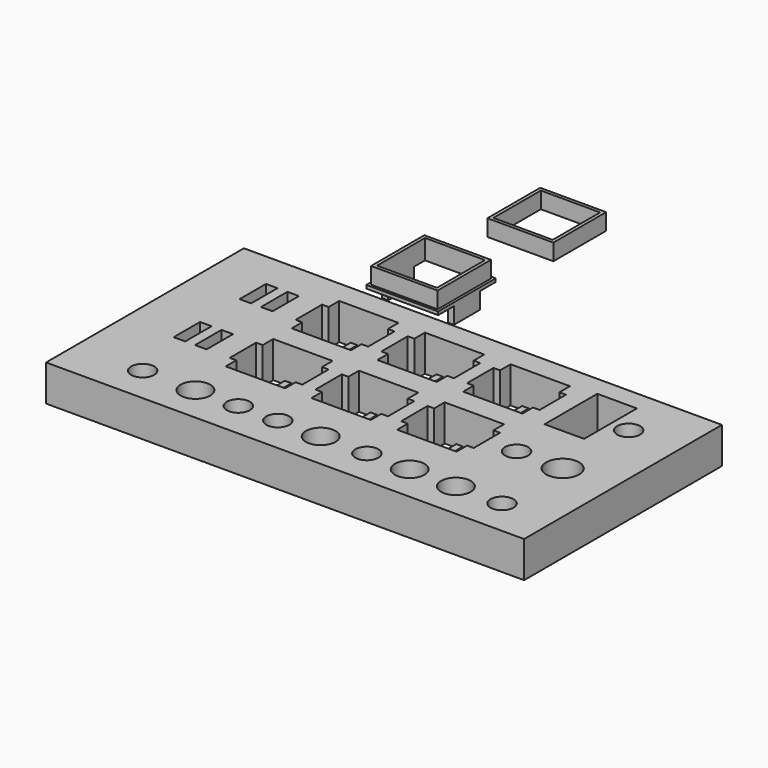
from build123d import *

# Parameters (mm, degrees)
F0_W      = 145
F0_H      = 75
F0_R      = 3.5
F0_R_2    = 4.5
F0_R_3    = 5
F0_W_2    = 12
F0_H_2    = 20
F0_W_3    = 3
F0_H_3    = 10
F1_DEPTH  = 1
F2_DEPTH  = 10
F3_W      = 18
F3_H      = 18
F4_DEPTH  = 10
F5_W      = 2
F5_H      = 10
F6_DEPTH  = 10
F8_DEPTH  = 5
F7_W      = 1.8
F7_H      = 9.8
F9_DEPTH  = 1
F10_DEPTH = 5
F11_W     = 20.2
F11_H     = 20.2
F11_W_2   = 18.2
F11_H_2   = 18.2
F12_DEPTH = 5


with BuildPart() as f1:
    # F0 (on Top) → F1 (new body)
    with BuildSketch(Plane.XY):
        with Locations((-82.504784634, -17.5405644029)):
            Rectangle(F0_W, F0_H)
        with Locations((-134.504784634, -44.0405644029)):
            Circle(F0_R, mode=Mode.SUBTRACT)
        with Locations((-118.504784634, -44.0405644029)):
            Circle(F0_R_2, mode=Mode.SUBTRACT)
        with Locations((-105.504784634, -44.0405644029)):
            Circle(F0_R, mode=Mode.SUBTRACT)
        with Locations((-93.504784634, -44.0405644029)):
            Circle(F0_R, mode=Mode.SUBTRACT)
        Polygon((-129.504784634, -16.0405644029), (-129.504784634, -26.0405644029), (-133.004784634, -26.0405644029), (-136.004784634, -26.0405644029), (-139.504784634, -26.0405644029), (-139.504784634, -16.0405644029), (-136.004784634, -16.0405644029), (-133.004784634, -16.0405644029), align=None, mode=Mode.SUBTRACT)
        Polygon((-102.504784634, -22.0405644029), (-102.504784634, -30.0405644029), (-105.9770819313, -30.0405644029), (-107.9770819313, -30.0405644029), (-114.9770819313, -30.0405644029), (-116.9770819313, -30.0405644029), (-120.504784634, -30.0405644029), (-120.504784634, -22.0405644029), (-120.504784634, -20.0405644029), (-120.504784634, -12.0405644029), (-116.9770819313, -12.0405644029), (-114.9770819313, -12.0405644029), (-107.9770819313, -12.0405644029), (-105.9770819313, -12.0405644029), (-102.504784634, -12.0405644029), (-102.504784634, -20.0405644029), align=None, mode=Mode.SUBTRACT)
        Polygon((-76.504784634, -12.0405644029), (-76.504784634, -20.0405644029), (-76.504784634, -22.0405644029), (-76.504784634, -30.0405644029), (-79.9770819313, -30.0405644029), (-81.9770819313, -30.0405644029), (-88.9770819313, -30.0405644029), (-90.9770819313, -30.0405644029), (-94.504784634, -30.0405644029), (-94.504784634, -22.0405644029), (-94.504784634, -20.0405644029), (-94.504784634, -12.0405644029), (-90.9770819313, -12.0405644029), (-88.9770819313, -12.0405644029), (-81.9770819313, -12.0405644029), (-79.9770819313, -12.0405644029), align=None, mode=Mode.SUBTRACT)
        with Locations((-80.504784634, -44.0405644029)):
            Circle(F0_R_2, mode=Mode.SUBTRACT)
        with Locations((-66.504784634, -44.0405644029)):
            Circle(F0_R, mode=Mode.SUBTRACT)
        with Locations((-53.504784634, -44.0405644029)):
            Circle(F0_R_2, mode=Mode.SUBTRACT)
        with Locations((-39.504784634, -44.0405644029)):
            Circle(F0_R_2, mode=Mode.SUBTRACT)
        with Locations((-25.504784634, -44.0405644029)):
            Circle(F0_R, mode=Mode.SUBTRACT)
        Polygon((-50.504784634, -12.0405644029), (-50.504784634, -20.0405644029), (-50.504784634, -22.0405644029), (-50.504784634, -30.0405644029), (-53.9770819313, -30.0405644029), (-55.9770819313, -30.0405644029), (-62.9770819313, -30.0405644029), (-64.9770819313, -30.0405644029), (-68.504784634, -30.0405644029), (-68.504784634, -22.0405644029), (-68.504784634, -20.0405644029), (-68.504784634, -12.0405644029), (-64.9770819313, -12.0405644029), (-62.9770819313, -12.0405644029), (-55.9770819313, -12.0405644029), (-53.9770819313, -12.0405644029), align=None, mode=Mode.SUBTRACT)
        with Locations((-39.504784634, -21.0405644029)):
            Circle(F0_R, mode=Mode.SUBTRACT)
        with Locations((-25.504784634, -21.0405644029)):
            Circle(F0_R_3, mode=Mode.SUBTRACT)
        Polygon((-129.504784634, 8.9594355971), (-129.504784634, -1.0405644029), (-133.004784634, -1.0405644029), (-136.004784634, -1.0405644029), (-139.504784634, -1.0405644029), (-139.504784634, 8.9594355971), (-136.004784634, 8.9594355971), (-133.004784634, 8.9594355971), align=None, mode=Mode.SUBTRACT)
        Polygon((-102.504784634, 2.9594355971), (-102.504784634, -5.0405644029), (-106.004784634, -5.0405644029), (-108.004784634, -5.0405644029), (-115.004784634, -5.0405644029), (-117.004784634, -5.0405644029), (-120.504784634, -5.0405644029), (-120.504784634, 2.9594355971), (-120.504784634, 4.9594355971), (-120.504784634, 12.9594355971), (-117.004784634, 12.9594355971), (-115.004784634, 12.9594355971), (-108.004784634, 12.9594355971), (-106.004784634, 12.9594355971), (-102.504784634, 12.9594355971), (-102.504784634, 4.9594355971), align=None, mode=Mode.SUBTRACT)
        Polygon((-94.504784634, 12.9594355971), (-91.004784634, 12.9594355971), (-89.004784634, 12.9594355971), (-82.004784634, 12.9594355971), (-80.004784634, 12.9594355971), (-76.504784634, 12.9594355971), (-76.504784634, 4.9594355971), (-76.504784634, 2.9594355971), (-76.504784634, -5.0405644029), (-80.004784634, -5.0405644029), (-82.004784634, -5.0405644029), (-89.004784634, -5.0405644029), (-91.004784634, -5.0405644029), (-94.504784634, -5.0405644029), (-94.504784634, 2.9594355971), (-94.504784634, 4.9594355971), align=None, mode=Mode.SUBTRACT)
        Polygon((-68.504784634, 12.9594355971), (-65.004784634, 12.9594355971), (-63.004784634, 12.9594355971), (-56.004784634, 12.9594355971), (-54.004784634, 12.9594355971), (-50.504784634, 12.9594355971), (-50.504784634, 4.9594355971), (-50.504784634, 2.9594355971), (-50.504784634, -5.0405644029), (-54.004784634, -5.0405644029), (-56.004784634, -5.0405644029), (-63.004784634, -5.0405644029), (-65.004784634, -5.0405644029), (-68.504784634, -5.0405644029), (-68.504784634, 2.9594355971), (-68.504784634, 4.9594355971), align=None, mode=Mode.SUBTRACT)
        with Locations((-37.004784634, 3.9594355971)):
            Rectangle(F0_W_2, F0_H_2, mode=Mode.SUBTRACT)
        with Locations((-25.504784634, 3.9594355971)):
            Circle(F0_R, mode=Mode.SUBTRACT)
        Polygon((-108.004784634, -5.0405644029), (-106.004784634, -5.0405644029), (-106.004784634, 2.9594355971), (-102.504784634, 2.9594355971), (-102.504784634, 4.9594355971), (-106.004784634, 4.9594355971), (-106.004784634, 12.9594355971), (-108.004784634, 12.9594355971), (-108.004784634, 4.9594355971), (-115.004784634, 4.9594355971), (-115.004784634, 12.9594355971), (-117.004784634, 12.9594355971), (-117.004784634, 4.9594355971), (-120.504784634, 4.9594355971), (-120.504784634, 2.9594355971), (-117.004784634, 2.9594355971), (-117.004784634, -5.0405644029), (-115.004784634, -5.0405644029), (-115.004784634, 2.9594355971), (-108.004784634, 2.9594355971), align=None)
        Polygon((-107.9770819313, -30.0405644029), (-105.9770819313, -30.0405644029), (-105.9770819313, -22.0405644029), (-102.504784634, -22.0405644029), (-102.504784634, -20.0405644029), (-105.9770819313, -20.0405644029), (-105.9770819313, -12.0405644029), (-107.9770819313, -12.0405644029), (-107.9770819313, -20.0405644029), (-114.9770819313, -20.0405644029), (-114.9770819313, -12.0405644029), (-116.9770819313, -12.0405644029), (-116.9770819313, -20.0405644029), (-120.504784634, -20.0405644029), (-120.504784634, -22.0405644029), (-116.9770819313, -22.0405644029), (-116.9770819313, -30.0405644029), (-114.9770819313, -30.0405644029), (-114.9770819313, -22.0405644029), (-107.9770819313, -22.0405644029), align=None)
        Polygon((-91.004784634, 12.9594355971), (-91.004784634, 4.9594355971), (-94.504784634, 4.9594355971), (-94.504784634, 2.9594355971), (-91.004784634, 2.9594355971), (-91.004784634, -5.0405644029), (-89.004784634, -5.0405644029), (-89.004784634, 2.9594355971), (-82.004784634, 2.9594355971), (-82.004784634, -5.0405644029), (-80.004784634, -5.0405644029), (-80.004784634, 2.9594355971), (-76.504784634, 2.9594355971), (-76.504784634, 4.9594355971), (-80.004784634, 4.9594355971), (-80.004784634, 12.9594355971), (-82.004784634, 12.9594355971), (-82.004784634, 4.9594355971), (-89.004784634, 4.9594355971), (-89.004784634, 12.9594355971), align=None)
        Polygon((-65.004784634, 12.9594355971), (-65.004784634, 4.9594355971), (-68.504784634, 4.9594355971), (-68.504784634, 2.9594355971), (-65.004784634, 2.9594355971), (-65.004784634, -5.0405644029), (-63.004784634, -5.0405644029), (-63.004784634, 2.9594355971), (-56.004784634, 2.9594355971), (-56.004784634, -5.0405644029), (-54.004784634, -5.0405644029), (-54.004784634, 2.9594355971), (-50.504784634, 2.9594355971), (-50.504784634, 4.9594355971), (-54.004784634, 4.9594355971), (-54.004784634, 12.9594355971), (-56.004784634, 12.9594355971), (-56.004784634, 4.9594355971), (-63.004784634, 4.9594355971), (-63.004784634, 12.9594355971), align=None)
        Polygon((-50.504784634, -22.0405644029), (-50.504784634, -20.0405644029), (-53.9770819313, -20.0405644029), (-53.9770819313, -12.0405644029), (-55.9770819313, -12.0405644029), (-55.9770819313, -20.0405644029), (-62.9770819313, -20.0405644029), (-62.9770819313, -12.0405644029), (-64.9770819313, -12.0405644029), (-64.9770819313, -20.0405644029), (-68.504784634, -20.0405644029), (-68.504784634, -22.0405644029), (-64.9770819313, -22.0405644029), (-64.9770819313, -30.0405644029), (-62.9770819313, -30.0405644029), (-62.9770819313, -22.0405644029), (-55.9770819313, -22.0405644029), (-55.9770819313, -30.0405644029), (-53.9770819313, -30.0405644029), (-53.9770819313, -22.0405644029), align=None)
        Polygon((-76.504784634, -22.0405644029), (-76.504784634, -20.0405644029), (-79.9770819313, -20.0405644029), (-79.9770819313, -12.0405644029), (-81.9770819313, -12.0405644029), (-81.9770819313, -20.0405644029), (-88.9770819313, -20.0405644029), (-88.9770819313, -12.0405644029), (-90.9770819313, -12.0405644029), (-90.9770819313, -20.0405644029), (-94.504784634, -20.0405644029), (-94.504784634, -22.0405644029), (-90.9770819313, -22.0405644029), (-90.9770819313, -30.0405644029), (-88.9770819313, -30.0405644029), (-88.9770819313, -22.0405644029), (-81.9770819313, -22.0405644029), (-81.9770819313, -30.0405644029), (-79.9770819313, -30.0405644029), (-79.9770819313, -22.0405644029), align=None)
        with Locations((-134.504784634, 3.9594355971)):
            Rectangle(F0_W_3, F0_H_3)
        with Locations((-134.504784634, -21.0405644029)):
            Rectangle(F0_W_3, F0_H_3)
    extrude(amount=F1_DEPTH)

    # F2 (add): a face of the model
    f2_faces = [f1.faces().sort_by_distance(p)[0] for p in [
        (-82.504784634, 18.3269528253, 1),
    ]]
    extrude(f2_faces, amount=F2_DEPTH)

    # F3 (on face) → F4 (cut)
    with BuildSketch(Plane.XY.offset(11)):
        with Locations((-111.504784634, 3.9594355971)):
            Rectangle(F3_W, F3_H)
        with Locations((-111.504784634, -21.0405644029)):
            Rectangle(F3_W, F3_H)
        with Locations((-85.504784634, 3.9594355971)):
            Rectangle(F3_W, F3_H)
        with Locations((-85.504784634, -21.0405644029)):
            Rectangle(F3_W, F3_H)
        with Locations((-59.504784634, 3.9594355971)):
            Rectangle(F3_W, F3_H)
        with Locations((-59.504784634, -21.0405644029)):
            Rectangle(F3_W, F3_H)
    extrude(amount=-F4_DEPTH, mode=Mode.SUBTRACT)

    # F5 (on face) → F6 (cut)
    with BuildSketch(Plane.XY.offset(11)):
        with Locations((-121.504784634, 3.9594355971)):
            Rectangle(F5_W, F5_H)
        with Locations((-101.504784634, 3.9594355971)):
            Rectangle(F5_W, F5_H)
        with Locations((-75.504784634, 3.9594355971)):
            Rectangle(F5_W, F5_H)
        with Locations((-95.504784634, 3.9594355971)):
            Rectangle(F5_W, F5_H)
        with Locations((-49.504784634, 3.9594355971)):
            Rectangle(F5_W, F5_H)
        with Locations((-69.504784634, 3.9594355971)):
            Rectangle(F5_W, F5_H)
        with Locations((-121.504784634, -21.0405644029)):
            Rectangle(F5_W, F5_H)
        with Locations((-101.504784634, -21.0405644029)):
            Rectangle(F5_W, F5_H)
        with Locations((-95.504784634, -21.0405644029)):
            Rectangle(F5_W, F5_H)
        with Locations((-75.504784634, -21.0405644029)):
            Rectangle(F5_W, F5_H)
        with Locations((-69.504784634, -21.0405644029)):
            Rectangle(F5_W, F5_H)
        with Locations((-49.504784634, -21.0405644029)):
            Rectangle(F5_W, F5_H)
    extrude(amount=-F6_DEPTH, mode=Mode.SUBTRACT)


with BuildPart() as f8:
    # F7 (on Top) → F8 (new body)
    with BuildSketch(Plane.XY):
        Polygon((-107.7882362008, 82.0260888338), (-106.7882362008, 82.0260888338), (-106.7882362008, 92.0260888338), (-107.7882362008, 92.0260888338), (-107.7882362008, 87.5260888338), (-107.7882362008, 86.5260888338), align=None)
        Polygon((-107.7882362008, 92.0260888338), (-106.7882362008, 92.0260888338), (-106.7882362008, 97.0260888338), (-126.7882362008, 97.0260888338), (-126.7882362008, 92.0260888338), (-125.7882362008, 92.0260888338), (-125.7882362008, 96.0260888338), (-107.7882362008, 96.0260888338), align=None)
        Polygon((-126.7882362008, 77.0260888338), (-106.7882362008, 77.0260888338), (-106.7882362008, 82.0260888338), (-107.7882362008, 82.0260888338), (-107.7882362008, 78.0260888338), (-125.7882362008, 78.0260888338), (-125.7882362008, 82.0260888338), (-126.7882362008, 82.0260888338), align=None)
        Polygon((-126.7882362008, 92.0260888338), (-126.7882362008, 82.0260888338), (-125.7882362008, 82.0260888338), (-125.7882362008, 86.5260888338), (-125.7882362008, 87.5260888338), (-125.7882362008, 92.0260888338), align=None)
    extrude(amount=F8_DEPTH)


with BuildPart() as f9:
    # F7 (on Top) → F9 (new body)
    with BuildSketch(Plane.XY):
        Polygon((-132.6183355093, 38.3936729491), (-110.8183355093, 38.3936729491), (-110.8183355093, 44.3936729491), (-112.6183355093, 44.3936729491), (-112.6183355093, 40.1936729491), (-130.8183355093, 40.1936729491), (-130.8183355093, 44.3936729491), (-132.6183355093, 44.3936729491), align=None)
        with Locations((-111.7183355093, 49.2936729491)):
            Rectangle(F7_W, F7_H)
        with Locations((-131.7183355093, 49.2936729491)):
            Rectangle(F7_W, F7_H)
        Polygon((-112.6183355093, 54.1936729491), (-110.8183355093, 54.1936729491), (-110.8183355093, 60.1936729491), (-132.6183355093, 60.1936729491), (-132.6183355093, 54.1936729491), (-130.8183355093, 54.1936729491), (-130.8183355093, 58.3936729491), (-112.6183355093, 58.3936729491), align=None)
    extrude(amount=F9_DEPTH)

    # F7 (on Top) → F10 (join)
    with BuildSketch(Plane.XY):
        with Locations((-131.7183355093, 49.2936729491)):
            Rectangle(F7_W, F7_H)
        with Locations((-111.7183355093, 49.2936729491)):
            Rectangle(F7_W, F7_H)
    extrude(amount=-F10_DEPTH)

    # F11 (on face) → F12 (join)
    with BuildSketch(Plane.XY.offset(1)):
        with Locations((-121.7183355093, 49.2936729491)):
            Rectangle(F11_W, F11_H)
        with Locations((-121.7183355093, 49.2936729491)):
            Rectangle(F11_W_2, F11_H_2, mode=Mode.SUBTRACT)
    extrude(amount=F12_DEPTH)


solid = Compound([f1.part, f8.part, f9.part])
